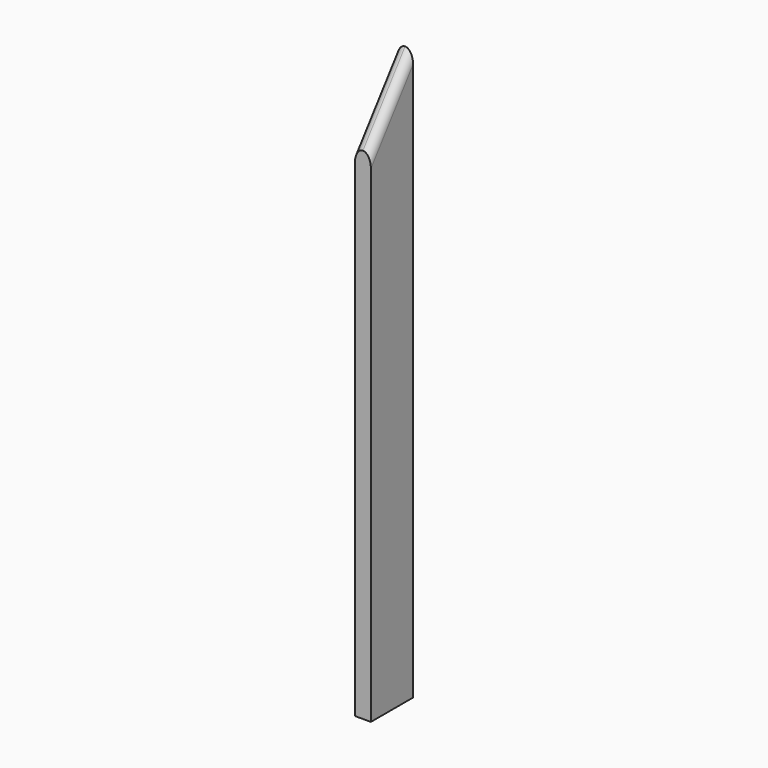
from build123d import *

# Parameters (mm, degrees)
F0_W     = 14.4847853028
F0_H     = 313
F1_DEPTH = 10
F2_R     = 4.99999


# Not quite as in the source:
# - a fillet or chamfer is up to 0.001 mm smaller than in the source, because OpenCascade refuses the exact size


with BuildPart() as f1:
    # F0 (on Right) → F1 (new body)
    with BuildSketch(Plane.YZ):
        with Locations((-49.3265521361, 156.5)):
            Rectangle(F0_W, F0_H)
        Polygon((-42.0841594847, 313), (-42.0841594847, 0), (-23.5623567487, 0), (-23.5623567487, 356.9950582001), (-56.5689447875, 313), align=None)
    extrude(amount=F1_DEPTH)

    # F2 (radius 5 in the source; OpenCascade refuses exactly that, so slightly less here)
    f2_edges = [f1.edges().sort_by_distance(p)[0] for p in [
        (10, -40.065651, 334.997529),
        (0, -40.065651, 334.997529),
    ]]
    fillet(f2_edges, radius=F2_R)


solid = f1.part
